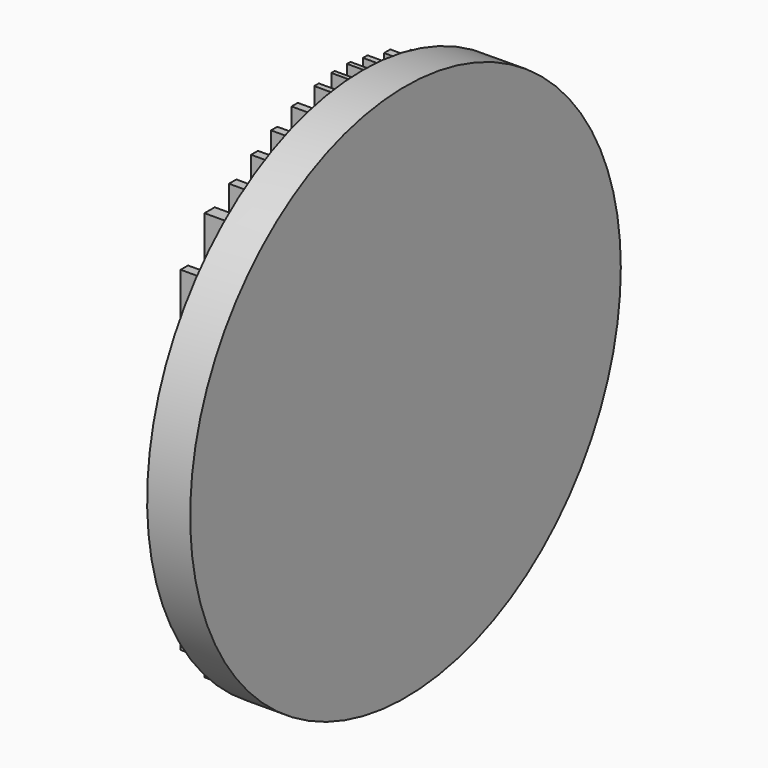
from build123d import *

# Parameters (mm, degrees)
F0_R        = 15.875
F1_DEPTH    = 2.54
F2_W        = 0.2515364613
F2_H        = 31.190475449
F2_W_2      = 0.335381832
F2_H_2      = 30.6035578251
F2_W_3      = 0.4611494951
F2_H_3      = 29.9327941611
F2_H_4      = 28.8428049535
F2_W_4      = 0.5030720495
F2_H_5      = 27.5432020426
F2_W_5      = 0.5449950695
F2_H_6      = 25.9082177654
F2_W_6      = 0.7546087727
F2_H_7      = 24.1055423394
F2_H_8      = 19.7455827147
F3_DEPTH    = 1.27
F4_T1_DEPTH = 8.9452554821


# Not quite as in the source:
# - a fillet or chamfer that OpenCascade refuses, or shapes differently, is made with other operations: its cross-section is extruded or revolved along the edge and cut away or added


with BuildPart() as f1:
    # F0 (on Right) → F1 (new body)
    with BuildSketch(Plane.YZ):
        Circle(F0_R)
    extrude(amount=F1_DEPTH)

    # F2 (on Right) → F3 (join)
    with BuildSketch(Plane.YZ):
        with Locations((-0.5812076997, 0.0161286443)):
            Rectangle(F2_W, F2_H)
        with Locations((-1.7969654873, 0.1418972388)):
            Rectangle(F2_W_2, F2_H_2)
        with Locations((-3.4109887201, 0.0999742188)):
            Rectangle(F2_W_3, F2_H_3)
        with Locations((-4.9202053342, 0.0161286443)):
            Rectangle(F2_W_3, F2_H_4)
        with Locations((-6.366537651, -0.0048326328)):
            Rectangle(F2_W_4, F2_H_5)
        with Locations((-7.9805608839, -0.0257934444)):
            Rectangle(F2_W_5, F2_H_6)
        with Locations((-9.6784294583, 0.0790129416)):
            Rectangle(F2_W_6, F2_H_7)
        with Locations((-11.5439891815, 0.0370899215)):
            Rectangle(F2_W_5, F2_H_8)
        with Locations((0.5812076997, 0.0161286443)):
            Rectangle(F2_W, F2_H)
        with Locations((11.5439891815, 0.0370899215)):
            Rectangle(F2_W_5, F2_H_8)
        with Locations((1.7969654873, 0.1418972388)):
            Rectangle(F2_W_2, F2_H_2)
        with Locations((3.4109887201, 0.0999742188)):
            Rectangle(F2_W_3, F2_H_3)
        with Locations((4.9202053342, 0.0161286443)):
            Rectangle(F2_W_3, F2_H_4)
        with Locations((9.6784294583, 0.0790129416)):
            Rectangle(F2_W_6, F2_H_7)
        with Locations((7.9805608839, -0.0257934444)):
            Rectangle(F2_W_5, F2_H_6)
        with Locations((6.366537651, -0.0048326328)):
            Rectangle(F2_W_4, F2_H_5)
    extrude(amount=-F3_DEPTH)

    # F4: fillet of radius 5.08 on 1 edges, made by hand

    # F4_s2 → F4_t1 (cut)
    with BuildSketch(Plane.XZ.offset(-20.2167471289)):
        with BuildLine():
            ThreePointArc((0, 9.9098812789), (-0.9419048812, 8.345828338), (-1.27, 6.5497771138))
            Line((-1.27, 6.5497771138), (-1.27, 9.9098812789))
            Line((-1.27, 9.9098812789), (0, 9.9098812789))
        make_face()
    extrude(amount=F4_T1_DEPTH, mode=Mode.SUBTRACT)


solid = f1.part
